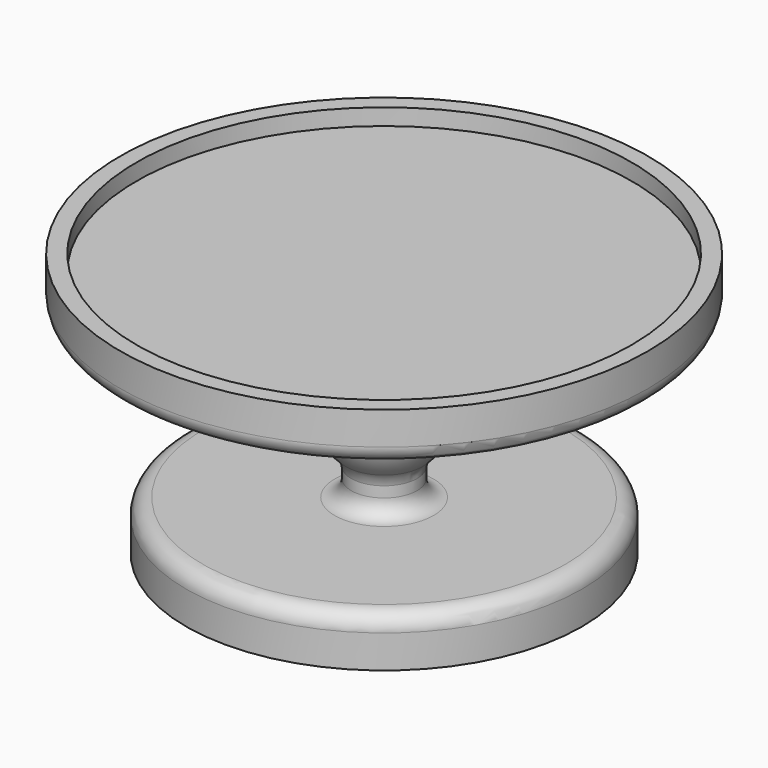
from build123d import *

# Parameters (mm, degrees)
F2_R = 3.175


# Not quite as in the source:
# - a feature names something its author has since deleted; it is built from what else it names


with BuildPart() as f1:
    # F0 (on Front) → F1 (revolve)
    with BuildSketch(Plane.XZ):
        Polygon((0, 6.35), (0, 0), (6.35, 0), (50.8, 0), (50.8, 9.525), (47.625, 9.525), (47.625, 6.35), align=None)
        Polygon((6.35, -31.75), (0, -31.75), (0, -41.275), (38.1, -41.275), (38.1, -31.75), align=None)
        with BuildLine():
            Line((6.35, 0), (0, 0))
            Line((0, 0), (0, -4.7625))
            ThreePointArc((0, -4.7625), (3.3277085246, -5.2724525596), (6.35, -6.7555067986))
            Line((6.35, -6.7555067986), (6.35, 0))
        make_face()
        with BuildLine():
            ThreePointArc((6.35, -24.9944932014), (3.3277085246, -26.4775474404), (0, -26.9875))
            Line((0, -26.9875), (0, -31.75))
            Line((0, -31.75), (6.35, -31.75))
            Line((6.35, -31.75), (6.35, -24.9944932014))
        make_face()
        with BuildLine():
            ThreePointArc((6.35, -6.7555067986), (3.3277085246, -5.2724525596), (0, -4.7625))
            Line((0, -4.7625), (0, -26.9875))
            ThreePointArc((0, -26.9875), (3.3277085246, -26.4775474404), (6.35, -24.9944932014))
            Line((6.35, -24.9944932014), (6.35, -6.7555067986))
        make_face()
        with BuildLine():
            ThreePointArc((11.1125, -15.875), (9.8501784565, -10.7309120706), (6.35, -6.7555067986))
            Line((6.35, -6.7555067986), (6.35, -24.9944932014))
            ThreePointArc((6.35, -24.9944932014), (9.8501784565, -21.0190879294), (11.1125, -15.875))
        make_face()
    revolve(axis=Axis((0, 0, 19.689680915), (0, 0, 1)))

    # F2
    f2_edges = [f1.edges().sort_by_distance(p)[0] for p in [
        (-6.35, 0, 0),
        (-6.35, 0, -6.755507),
        (11.1125, 0, -15.875),
        (6.35, 0, -3.377753),
        (-6.35, 0, -24.994493),
        (6.35, 0, -28.372247),
        (-6.35, 0, -31.75),
        (-50.8, 0, 0),
        (-38.1, 0, -31.75),
    ]]
    fillet(f2_edges, radius=F2_R)


solid = f1.part
